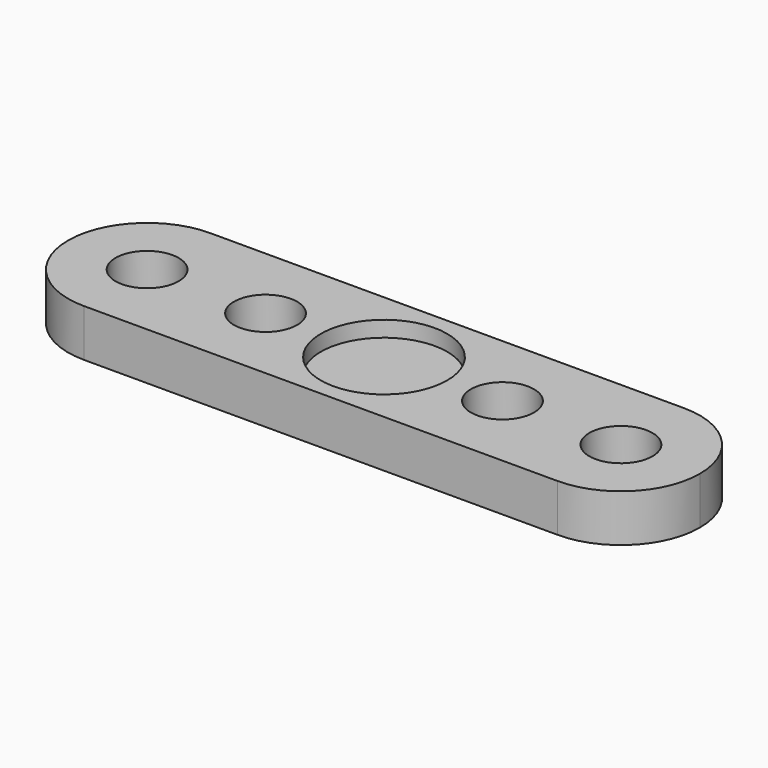
from build123d import *

# Parameters (mm, degrees)
F0_W     = 40
F0_H     = 10
F1_DEPTH = 3
F2_R     = 4
F3_DEPTH = 1
F4_R     = 2
F5_DEPTH = 25
F6_R     = 4.99999


# Not quite as in the source:
# - a fillet or chamfer is up to 0.001 mm smaller than in the source, because OpenCascade refuses the exact size


with BuildPart() as f1:
    # F0 (on Top) → F1 (new body)
    with BuildSketch(Plane.XY):
        Rectangle(F0_W, F0_H)
    extrude(amount=F1_DEPTH)

    # F2 (on face) → F3 (cut)
    with BuildSketch(Plane.XY.offset(3)):
        Circle(F2_R)
    extrude(amount=-F3_DEPTH, mode=Mode.SUBTRACT)

    # F4 (on Top) → F5 (cut)
    with BuildSketch(Plane.XY):
        with Locations((-7.5, 0)):
            Circle(F4_R)
        with Locations((7.5, 0)):
            Circle(F4_R)
        with Locations((-15, 0)):
            Circle(F4_R)
        with Locations((15, 0)):
            Circle(F4_R)
    extrude(amount=F5_DEPTH, mode=Mode.SUBTRACT)

    # F6 (radius 5 in the source; OpenCascade refuses exactly that, so slightly less here)
    f6_edges = [f1.edges().sort_by_distance(p)[0] for p in [
        (-20, -5, 1.5),
        (-20, 5, 1.5),
        (20, -5, 1.5),
        (20, 5, 1.5),
    ]]
    fillet(f6_edges, radius=F6_R)


solid = f1.part
